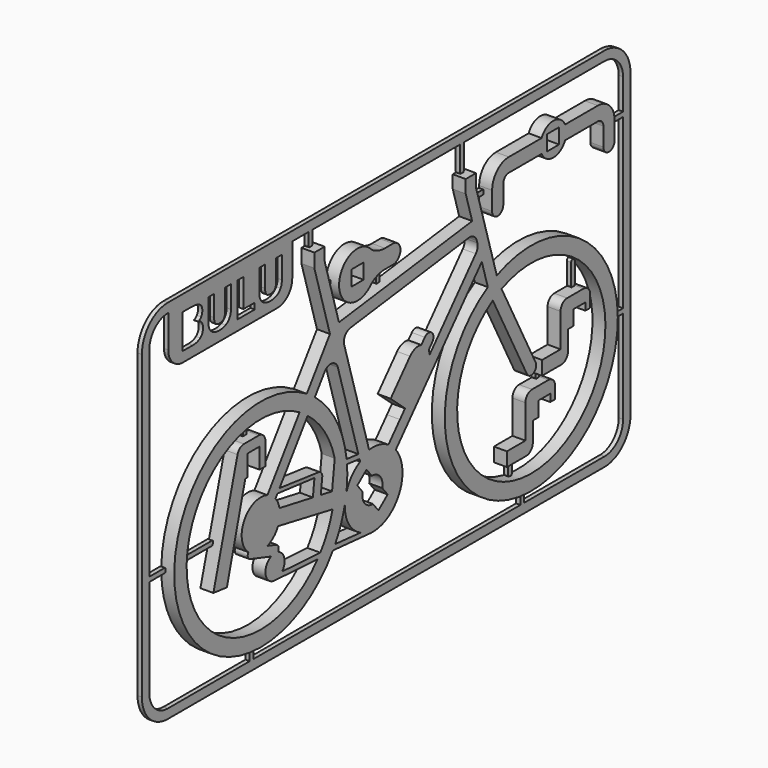
from build123d import *

# Parameters (mm, degrees)
F2_DEPTH = 2.8
F1_W     = 3.286
F1_H     = 3.286
F1_W_2   = 3.2
F1_H_2   = 3.2858568893
F3_DEPTH = 0.9333333333
F5_DEPTH = 0.9333333333
F7_DEPTH = 0.9333333333


# Not quite as in the source:
# - ends of sketch curves that miss each other by under 0.0002 mm in the source are joined
# - a feature names something its author has since deleted; it is built from what else it names


with BuildPart() as f2:
    # F1 (on Right) → F2 (new body)
    with BuildSketch(Plane.YZ):
        with BuildLine():
            Line((-32.7810810621, 40.0630099882), (-28.5785464468, 25.854345194))
            Line((-28.5785464468, 25.854345194), (-34.8295213879, 17.0517607704))
            ThreePointArc((-34.8295213879, 17.0517607704), (-70.0441528649, -7.6634310767), (-27.7561804721, -15.577871613))
            Line((-27.7561804721, -15.577871613), (-17.4309209468, -16.4342678025))
            ThreePointArc((-17.4309209468, -16.4342678025), (-17.421352009, -16.4349690955), (-17.4117713764, -16.4354866475))
            ThreePointArc((-17.4117713764, -16.4354866475), (-9.8783278177, -12.024945839), (-10.8100300989, -3.3452239002))
            Line((-10.8100300989, -3.3452239002), (12.3781786089, 22.9225390659))
            Line((12.3781786089, 22.9225390659), (13.9960358427, 17.4527707038))
            ThreePointArc((13.9960358427, 17.4527707038), (36.2440392418, -23.5369879191), (16.4146126558, 18.6758988393))
            Line((16.4146126558, 18.6758988393), (14.2536723845, 25.9817614853))
            ThreePointArc((14.2536723845, 25.9817614853), (14.2515405676, 25.989045047), (14.2493673209, 25.9963163545))
            Line((14.2493673209, 25.9963163545), (12.7777300944, 30.9717335764))
            Line((12.7777300944, 30.9717335764), (10.8173713638, 37.5995357396))
            Line((10.8173713638, 37.5995357396), (10.8173713638, 40.3995357399))
            Line((10.8173713638, 40.3995357399), (8.037018366, 40.3995357399))
            Line((8.037018366, 40.3995357399), (8.037018366, 37.5995357399))
            Line((8.037018366, 37.5995357399), (9.7773678827, 31.7155655707))
            Line((9.7773678827, 31.7155655707), (-26.1566620581, 27.0789083905))
            Line((-26.1566620581, 27.0789083905), (-30.0007321323, 40.2276701755))
            Line((-30.0007321323, 40.2276701755), (-30.0007321323, 43.0276701755))
            Line((-30.0007321323, 43.0276701755), (-32.7810810175, 43.0276701755))
            Line((-32.7810810175, 43.0276701755), (-32.7810810621, 40.0630099882))
        make_face()
        with BuildLine():
            ThreePointArc((-27.1589419206, -14.6239739066), (-25.6381564049, -11.5709515578), (-24.5785787783, -8.3288797973))
            ThreePointArc((-24.5785787783, -8.3288797973), (-23.4485868958, -12.4014570535), (-20.3032664054, -15.2245273988))
            Line((-20.3032664054, -15.2245273988), (-27.1589419206, -14.6239739066))
        make_face(mode=Mode.SUBTRACT)
        with BuildLine():
            Line((-36.7690909191, 14.3204708989), (-45.438959238, 2.1116157144))
            ThreePointArc((-45.438959238, 2.1116157144), (-51.679021575, -0.1114645339), (-50.5741858599, -6.6429116785))
            ThreePointArc((-50.5741858599, -6.6429116785), (-50.7001368643, -7.5358957288), (-50.0559554, -8.1670172786))
            Line((-50.0559554, -8.1670172786), (-44.4357401431, -9.9504751803))
            ThreePointArc((-44.4357401431, -9.9504751803), (-45.9475994843, -12.7053301629), (-43.682084094, -14.8830318549))
            Line((-43.682084094, -14.8830318549), (-43.4085644782, -14.8992046485))
            Line((-43.4085644782, -14.8992046485), (-31.9213599112, -15.5784253597))
            ThreePointArc((-31.9213599112, -15.5784253597), (-66.9726575865, -5.9191061127), (-36.7690909191, 14.3204708989))
        make_face(mode=Mode.SUBTRACT)
        with BuildLine():
            ThreePointArc((-45.417431414, -7.5410613439), (-43.7533998551, -6.5186996051), (-42.5893207169, -4.9505336974))
            Line((-42.5893207169, -4.9505336974), (-27.8742179451, -7.7233503042))
            ThreePointArc((-27.8742179451, -7.7233503042), (-29.1875288387, -11.3310895929), (-31.1661285889, -14.6213344633))
            Line((-31.1661285889, -14.6213344633), (-41.4453615912, -14.013539249))
            ThreePointArc((-41.4453615912, -14.013539249), (-40.8757428579, -11.7304415251), (-42.3931878811, -9.9320085072))
            Line((-42.3931878811, -9.9320085072), (-42.3931878811, -9.2324187691))
            ThreePointArc((-42.3931878811, -9.2324187691), (-42.5861622295, -8.6419628585), (-43.0905932927, -8.2794348124))
            Line((-43.0905932927, -8.2794348124), (-45.417431414, -7.5410613439))
        make_face(mode=Mode.SUBTRACT)
        with BuildLine():
            Line((-15.5088098858, -12.9576973057), (-16.9709924298, -11.149063212))
            ThreePointArc((-16.9709924298, -11.149063212), (-19.2224479888, -10.1072740955), (-19.7694541503, -7.6875301098))
            Line((-19.7694541503, -7.6875301098), (-21.2014292566, -5.9162608458))
            Line((-21.2014292566, -5.9162608458), (-18.7129342238, -3.9044476159))
            Line((-18.7129342238, -3.9044476159), (-17.2809591175, -5.67571688))
            ThreePointArc((-17.2809591175, -5.67571688), (-15.0295035586, -6.7175059964), (-14.4824973971, -9.1372499821))
            Line((-14.4824973971, -9.1372499821), (-13.0203148531, -10.9458840758))
            Line((-13.0203148531, -10.9458840758), (-15.5088098858, -12.9576973057))
        make_face(mode=Mode.SUBTRACT)
        with BuildLine():
            ThreePointArc((-20.4284332347, -1.7008787129), (-22.713034199, -3.5049348102), (-24.1327228009, -6.0462935497))
            ThreePointArc((-24.1327228009, -6.0462935497), (-23.9042746908, -3.4009611929), (-23.9777551737, -0.7467998497))
            Line((-23.9777551737, -0.7467998497), (-20.6010095051, -1.1174049345))
            Line((-20.6010095051, -1.1174049345), (-20.4284332347, -1.7008787129))
        make_face(mode=Mode.SUBTRACT)
        with BuildLine():
            ThreePointArc((-42.1876674295, -1.6755199445), (-42.5889328041, -0.4877747618), (-43.2651398515, 0.5679224243))
            Line((-43.2651398515, 0.5679224243), (-42.7367221094, 1.3120370351))
            Line((-42.7367221094, 1.3120370351), (-32.7536984043, 0.2163787562))
            Line((-32.7536984043, 0.2163787562), (-33.1812144267, -3.3188663768))
            Line((-33.1812144267, -3.3188663768), (-42.1876674295, -1.6755199445))
        make_face(mode=Mode.SUBTRACT)
        with BuildLine():
            Line((-31.6963693255, 0.8509632025), (-42.1651316758, 2.1169471643))
            Line((-42.1651316758, 2.1169471643), (-34.5952715328, 12.7767776084))
            ThreePointArc((-34.5952715328, 12.7767776084), (-29.9994401309, 7.8666759835), (-27.2914488726, 1.7105775773))
            Line((-27.2914488726, 1.7105775773), (-28.0136806178, -4.2617512446))
            Line((-28.0136806178, -4.2617512446), (-31.0443248868, -3.708770127))
            Line((-31.0443248868, -3.708770127), (-30.6536988323, -0.4785780739))
            ThreePointArc((-30.6536988323, -0.4785780739), (-30.8996770647, 0.402136694), (-31.6963693255, 0.8509632025))
        make_face(mode=Mode.SUBTRACT)
        with BuildLine():
            ThreePointArc((24.5326127574, -3.3329199604), (26.3299626073, -3.9019308276), (26.8989734744, -2.1045809777))
            Line((26.8989734744, -2.1045809777), (17.7069262182, 15.603641135))
            ThreePointArc((17.7069262182, 15.603641135), (34.9283354862, -20.4664558462), (15.3405655012, 14.3753021523))
            Line((15.3405655012, 14.3753021523), (24.5326127574, -3.3329199604))
        make_face(mode=Mode.SUBTRACT)
        with BuildLine():
            ThreePointArc((-29.9983734724, 19.2501011531), (-28.0396469956, 20.0648164886), (-26.4504948685, 18.6594816511))
            Line((-26.4504948685, 18.6594816511), (-20.9085424497, -0.0776477954))
            Line((-20.9085424497, -0.0776477954), (-24.0866021245, 0.2711510752))
            ThreePointArc((-24.0866021245, 0.2711510752), (-26.8907561473, 8.722170153), (-32.6557020014, 15.5080674802))
            Line((-32.6557020014, 15.5080674802), (-29.9983734724, 19.2501011531))
        make_face(mode=Mode.SUBTRACT)
        with BuildLine():
            Line((-18.0250834345, -0.4262562289), (-24.7288519992, 22.2389292241))
            ThreePointArc((-24.7288519992, 22.2389292241), (-24.4867438443, 23.8976541842), (-23.0672336955, 24.7892683327))
            Line((-23.0672336955, 24.7892683327), (8.8532049047, 28.9080418475))
            ThreePointArc((8.8532049047, 28.9080418475), (10.2006691115, 28.6002630517), (11.0266106326, 27.4920175106))
            Line((11.0266106326, 27.4920175106), (11.1717955661, 27.0011658215))
            ThreePointArc((11.1717955661, 27.0011658215), (11.2066686934, 26.0018903312), (10.7533788193, 25.1106575162))
            Line((10.7533788193, 25.1106575162), (-1.7245508843, 10.9755725718))
            ThreePointArc((-1.7245508843, 10.9755725718), (-1.7897327542, 11.4952481661), (-1.9443174541, 11.9956629641))
            Line((-1.9443174541, 11.9956629641), (-0.9945827645, 13.0715289795))
            ThreePointArc((-0.9945827646, 13.0715289795), (-1.1117489129, 14.9531537943), (-2.9933737277, 14.8359876459))
            Line((-2.9933737277, 14.8359876459), (-3.9431084172, 13.7601216304))
            ThreePointArc((-3.9431084172, 13.7601216304), (-5.5866841115, 13.7356227774), (-6.9705428385, 12.8485623057))
            Line((-6.9705428385, 12.8485623057), (-12.2077076552, 6.9158658319))
            Line((-12.2077076552, 6.9158658319), (-8.3300521573, 3.4928151103))
            Line((-8.3300521573, 3.4928151103), (-9.6983886135, 1.9427541226))
            Line((-9.6983886135, 1.9427541226), (-12.8088210603, -1.5807652347))
            ThreePointArc((-12.8088210603, -1.5807652347), (-15.3182270596, -0.5574540272), (-18.0250834345, -0.4262562289))
        make_face(mode=Mode.SUBTRACT)
    extrude(amount=F2_DEPTH)



with BuildPart() as f2b:
    # F1 (on Right) → F2, piece 2 (new body)
    with BuildSketch(Plane.YZ):
        with BuildLine():
            Line((26.1350085661, -17.0272199881), (26.1350085661, -12.8250569627))
            Line((26.1350085661, -12.8250569627), (27.6350085661, -12.8250569627))
            Line((27.6350085661, -12.8250569627), (27.6350085661, -9.6250569627))
            Line((27.6350085661, -9.6250569627), (30.8350085661, -9.6250569627))
            Line((30.8350085661, -9.6250569627), (30.8350085661, -11.2250569627))
            Line((30.8350085661, -11.2250569627), (32.1350085661, -11.2250569627))
            Line((32.1350085661, -11.2250569627), (32.1350085661, -8.6228939372))
            ThreePointArc((32.1350085661, -8.6228939372), (31.6084343077, -7.351631221), (30.3371715916, -6.8250569627))
            Line((30.3371715916, -6.8250569627), (26.1350085661, -6.8250569627))
            Line((26.1350085661, -6.8250569627), (25.9328455406, -6.8250569627))
            ThreePointArc((25.9328455406, -6.8250569627), (24.6615828245, -7.351631221), (24.1350085661, -8.6228939372))
            Line((24.1350085661, -8.6228939372), (24.1350085661, -15.8250569627))
            Line((24.1350085661, -15.8250569627), (19.1350085661, -15.8250569627))
            Line((19.1350085661, -15.8250569627), (19.1350085661, -18.8250569627))
            Line((19.1350085661, -18.8250569627), (24.3371715916, -18.8250569627))
            ThreePointArc((24.3371715916, -18.8250569627), (25.6084343077, -18.2984827043), (26.1350085661, -17.0272199881))
        make_face()
    extrude(amount=F2_DEPTH)


with BuildPart() as f2c:
    # F1 (on Right) → F2, piece 3 (new body)
    with BuildSketch(Plane.YZ):
        with BuildLine():
            Line((-47.7713023129, 14.3973374015), (-51.7613397022, 14.3973374015))
            ThreePointArc((-51.7613397022, 14.3973374015), (-52.8518038089, 14.0305013357), (-53.496568146, 13.077632186))
            Line((-53.496568146, 13.077632186), (-60.0158057756, -10.5528221893))
            Line((-60.0158057756, -10.5528221893), (-56.367214369, -10.9714387513))
            Line((-56.367214369, -10.9714387513), (-51.4058386912, 7.6636058447))
            Line((-51.4058386912, 7.6636058447), (-50.7571436434, 7.6636058447))
            Line((-50.7571436434, 7.6636058447), (-50.7571436434, 12.2000958209))
            Line((-50.7571436434, 12.2000958209), (-47.5571436434, 12.2000958209))
            Line((-47.5571436434, 12.2000958209), (-47.5571436434, 7.799523944))
            Line((-47.5571436434, 7.799523944), (-45.9734653383, 7.799523944))
            Line((-45.9734653383, 7.799523944), (-45.9734653383, 12.599500427))
            ThreePointArc((-45.9734653383, 12.599500427), (-46.5000395967, 13.8707631432), (-47.7713023129, 14.3973374015))
        make_face()
    extrude(amount=F2_DEPTH)


with BuildPart() as f2d:
    # F1 (on Right) → F2, piece 4 (new body)
    with BuildSketch(Plane.YZ):
        with BuildLine():
            ThreePointArc((-11.5660707645, 32.1164598398), (-9.5660707645, 34.1164598398), (-11.5660707645, 36.1164598398))
            Line((-11.5660707645, 36.1164598398), (-13.7510611544, 36.1164598398))
            ThreePointArc((-13.7510611544, 36.1164598398), (-15.6803701734, 36.4351072976), (-17.4047560543, 37.35720427))
            ThreePointArc((-17.4047560543, 37.35720427), (-26.1140103212, 34.1164598398), (-17.4047560543, 30.8757154096))
            ThreePointArc((-17.4047560543, 30.8757154096), (-15.6803701734, 31.7978123821), (-13.7510611544, 32.1164598398))
            Line((-13.7510611544, 32.1164598398), (-11.5660707645, 32.1164598398))
        make_face()
        with Locations((-21.1564369343, 34.1164598398)):
            Rectangle(F1_W, F1_H, mode=Mode.SUBTRACT)
    extrude(amount=F2_DEPTH)


with BuildPart() as f2e:
    # F1 (on Right) → F2, piece 5 (new body)
    with BuildSketch(Plane.YZ):
        with BuildLine():
            ThreePointArc((15.1628487238, 31.3657282359), (16.6628487238, 29.8657282359), (18.1628487238, 31.3657282359))
            Line((18.1628487238, 31.3657282359), (18.1628487238, 35.3657282359))
            ThreePointArc((18.1628487238, 35.3657282359), (18.602188552, 36.4263884077), (19.6628487238, 36.8657282359))
            Line((19.6628487238, 36.8657282359), (28.5005710636, 36.8657282359))
            ThreePointArc((28.5005710636, 36.8657282359), (31.6628487238, 34.8657282359), (34.825126384, 36.8657282359))
            Line((34.825126384, 36.8657282359), (43.6628487238, 36.8657282359))
            ThreePointArc((43.6628487238, 36.8657282359), (44.7235088956, 36.4263884077), (45.1628487238, 35.3657282359))
            Line((45.1628487238, 35.3657282359), (45.1628487238, 31.3657282359))
            ThreePointArc((45.1628487238, 31.3657282359), (46.6628487238, 29.8657282359), (48.1628487238, 31.3657282359))
            Line((48.1628487238, 31.3657282359), (48.1628487238, 35.3657282359))
            ThreePointArc((48.1628487238, 35.3657282359), (46.8448292391, 38.5477087513), (43.6628487238, 39.8657282359))
            Line((43.6628487238, 39.8657282359), (34.825126384, 39.8657282359))
            ThreePointArc((34.825126384, 39.8657282359), (31.6628487238, 41.8657282359), (28.5005710636, 39.8657282359))
            Line((28.5005710636, 39.8657282359), (19.6628487238, 39.8657282359))
            ThreePointArc((19.6628487238, 39.8657282359), (16.4808682084, 38.5477087513), (15.1628487238, 35.3657282359))
            Line((15.1628487238, 35.3657282359), (15.1628487238, 31.3657282359))
        make_face()
        with Locations((31.6199202791, 38.3657282359)):
            Rectangle(F1_W_2, F1_H_2, mode=Mode.SUBTRACT)
    extrude(amount=F2_DEPTH)


with BuildPart() as f2f:
    # F1 (on Right) → F2, piece 6 (new body)
    with BuildSketch(Plane.YZ):
        with BuildLine():
            Line((39.8146519543, 6.6714825634), (35.6124889288, 6.6714825634))
            Line((35.6124889288, 6.6714825634), (35.4103259033, 6.6714825634))
            ThreePointArc((35.4103259033, 6.6714825634), (34.1390631872, 6.144908305), (33.6124889288, 4.8736455889))
            Line((33.6124889288, 4.8736455889), (33.6124889288, -2.3285174366))
            Line((33.6124889288, -2.3285174366), (28.6124889288, -2.3285174366))
            Line((28.6124889288, -2.3285174366), (28.6124889288, -5.3285174366))
            Line((28.6124889288, -5.3285174366), (33.8146519543, -5.3285174366))
            ThreePointArc((33.8146519543, -5.3285174366), (35.0859146704, -4.8019431782), (35.6124889288, -3.5306804621))
            Line((35.6124889288, -3.5306804621), (35.6124889288, 0.6714825634))
            Line((35.6124889288, 0.6714825634), (37.1124889288, 0.6714825634))
            Line((37.1124889288, 0.6714825634), (37.1124889288, 3.8714825634))
            Line((37.1124889288, 3.8714825634), (40.3124889288, 3.8714825634))
            Line((40.3124889288, 3.8714825634), (40.3124889288, 2.2714825634))
            Line((40.3124889288, 2.2714825634), (41.6124889288, 2.2714825634))
            Line((41.6124889288, 2.2714825634), (41.6124889288, 4.8736455889))
            ThreePointArc((41.6124889288, 4.8736455889), (41.0859146704, 6.144908305), (39.8146519543, 6.6714825634))
        make_face()
    extrude(amount=F2_DEPTH)


with BuildPart() as f3:
    # F1 (on Right) → F3 (new body)
    with BuildSketch(Plane.YZ):
        with BuildLine():
            ThreePointArc((-76.9647278786, -24.0477662427), (-74.9144753469, -28.9975137111), (-69.9647278786, -31.0477662427))
            Line((-69.9647278786, -31.0477662427), (47.795983851, -31.0477662427))
            ThreePointArc((47.795983851, -31.0477662427), (52.7457313193, -28.9975137111), (54.795983851, -24.0477662427))
            Line((54.795983851, -24.0477662427), (54.795983851, 41.0276701755))
            ThreePointArc((54.795983851, 41.0276701755), (52.7457313193, 45.9774176438), (47.795983851, 48.0276701755))
            Line((47.795983851, 48.0276701755), (-69.9647278786, 48.0276701755))
            ThreePointArc((-69.9647278786, 48.0276701755), (-74.9144753469, 45.9774176438), (-76.9647278786, 41.0276701755))
            Line((-76.9647278786, 41.0276701755), (-76.9647278786, -24.0477662427))
        make_face()
        with BuildLine():
            Line((47.795983851, -29.0477662427), (-69.9647278786, -29.0477662427))
            ThreePointArc((-69.9647278786, -29.0477662427), (-73.5002617845, -27.5833001487), (-74.9647278786, -24.0477662427))
            Line((-74.9647278786, -24.0477662427), (-74.9647278786, 41.0276701755))
            ThreePointArc((-74.9647278786, 41.0276701755), (-73.5002617845, 44.5632040814), (-69.9647278786, 46.0276701755))
            Line((-69.9647278786, 46.0276701755), (-64.4556283951, 46.0276701755))
            Line((-64.4556283951, 46.0276701755), (-38.3469462395, 46.0276701755))
            Line((-38.3469462395, 46.0276701755), (47.795983851, 46.0276701755))
            ThreePointArc((47.795983851, 46.0276701755), (51.3315177569, 44.5632040814), (52.795983851, 41.0276701755))
            Line((52.795983851, 41.0276701755), (52.795983851, -24.0477662427))
            ThreePointArc((52.795983851, -24.0477662427), (51.3315177569, -27.5833001487), (47.795983851, -29.0477662427))
        make_face(mode=Mode.SUBTRACT)
    extrude(amount=F3_DEPTH)


with BuildPart() as f2_1:
    add(f2.part)

    add(f2b.part)  # F5 merges F2b

    add(f2c.part)  # F5 merges F2c

    add(f2d.part)  # F5 merges F2d

    add(f2e.part)  # F5 merges F2e

    add(f2f.part)  # F5 merges F2f

    add(f3.part)  # F5 merges F3
    # F4 (on Right) → F5 (join)
    with BuildSketch(Plane.YZ):
        with BuildLine():
            ThreePointArc((-49.7433960476, 14.0407793284), (-49.2433960476, 13.5407793284), (-48.7433960476, 14.0407793284))
            Line((-48.7433960476, 14.0407793284), (-48.7433960476, 16.7634686467))
            ThreePointArc((-48.7433960476, 16.7634686467), (-49.2433960476, 17.2634686467), (-49.7433960476, 16.7634686467))
            Line((-49.7433960476, 16.7634686467), (-49.7433960476, 14.0407793284))
        make_face()
        with BuildLine():
            ThreePointArc((-66.8206203722, -2.0058723694), (-67.3206203722, -2.5058723694), (-66.8206203722, -3.0058723694))
            Line((-66.8206203722, -3.0058723694), (-58.1512004137, -3.0058723694))
            ThreePointArc((-58.1512004137, -3.0058723694), (-57.6512004137, -2.5058723694), (-58.1512004137, -2.0058723694))
            Line((-58.1512004137, -2.0058723694), (-66.8206203722, -2.0058723694))
        make_face()
        with BuildLine():
            ThreePointArc((-70.9232541835, -3.0058723694), (-70.4232541835, -2.5058723694), (-70.9232541835, -2.0058723694))
            Line((-70.9232541835, -2.0058723694), (-74.9647278786, -2.0058723694))
            ThreePointArc((-74.9647278786, -2.0058723694), (-75.4647278786, -2.5058723694), (-74.9647278786, -3.0058723694))
            Line((-74.9647278786, -3.0058723694), (-70.9232541835, -3.0058723694))
        make_face()
        with BuildLine():
            ThreePointArc((-31.9633883536, 43.3622263372), (-31.4633883536, 42.8622263372), (-30.9633883536, 43.3622263372))
            Line((-30.9633883536, 43.3622263372), (-30.9633883536, 46.4626848698))
            ThreePointArc((-30.9633883536, 46.4626848698), (-31.4633883536, 46.9626848698), (-31.9633883536, 46.4626848698))
            Line((-31.9633883536, 46.4626848698), (-31.9633883536, 43.3622263372))
        make_face()
        with BuildLine():
            ThreePointArc((-27.9091558336, 34.6210477054), (-28.4091558336, 34.1210477054), (-27.9091558336, 33.6210477054))
            Line((-27.9091558336, 33.6210477054), (-26.4964278766, 33.6210477054))
            ThreePointArc((-26.4964278766, 33.6210477054), (-25.9964278766, 34.1210477054), (-26.4964278766, 34.6210477054))
            Line((-26.4964278766, 34.6210477054), (-27.9091558336, 34.6210477054))
        make_face()
        with BuildLine():
            Line((-13.8486790583, 31.6781923175), (-13.8486790583, 29.1007384658))
            ThreePointArc((-13.8486790583, 29.1007384658), (-13.3486790583, 28.6007384658), (-12.8486790583, 29.1007384658))
            Line((-12.8486790583, 29.1007384658), (-12.8486790583, 31.6781923175))
            ThreePointArc((-12.8486790583, 31.6781923175), (-13.3486790583, 32.1781923175), (-13.8486790583, 31.6781923175))
        make_face()
        with BuildLine():
            Line((8.8458192423, 46.0585150868), (8.8458192423, 40.6653936952))
            ThreePointArc((8.8458192423, 40.6653936952), (9.3458192423, 40.1653936952), (9.8458192423, 40.6653936952))
            Line((9.8458192423, 40.6653936952), (9.8458192423, 46.0585150868))
            ThreePointArc((9.8458192423, 46.0585150868), (9.3458192423, 46.5585150868), (8.8458192423, 46.0585150868))
        make_face()
        with BuildLine():
            ThreePointArc((11.9448483718, 34.9700198621), (11.4448483718, 34.4700198621), (11.9448483718, 33.9700198621))
            Line((11.9448483718, 33.9700198621), (14.8754121757, 33.9700198621))
            ThreePointArc((14.8754121757, 33.9700198621), (15.3754121757, 34.4700198621), (14.8754121757, 34.9700198621))
            Line((14.8754121757, 34.9700198621), (11.9448483718, 34.9700198621))
        make_face()
        with BuildLine():
            ThreePointArc((48.4550757053, 34.3975656778), (47.9550757053, 33.8975656778), (48.4550757053, 33.3975656778))
            Line((48.4550757053, 33.3975656778), (52.9664561174, 33.3975656778))
            ThreePointArc((52.9664561174, 33.3975656778), (53.4664561174, 33.8975656778), (52.9664561174, 34.3975656778))
            Line((52.9664561174, 34.3975656778), (48.4550757053, 34.3975656778))
        make_face()
        with BuildLine():
            Line((38.7966382205, 11.4560816437), (38.7966382205, 6.9804331288))
            ThreePointArc((38.7966382205, 6.9804331288), (39.2966382205, 6.4804331288), (39.7966382205, 6.9804331288))
            Line((39.7966382205, 6.9804331288), (39.7966382205, 11.4560816437))
            ThreePointArc((39.7966382205, 11.4560816437), (39.2966382205, 11.9560816437), (38.7966382205, 11.4560816437))
        make_face()
        with BuildLine():
            Line((49.2580496178, -3.9376585865), (53.1618170887, -3.9376585865))
            ThreePointArc((53.1618170887, -3.9376585865), (53.6618170887, -3.4376585865), (53.1618170887, -2.9376585865))
            Line((53.1618170887, -2.9376585865), (49.2580496178, -2.9376585865))
            ThreePointArc((49.2580496178, -2.9376585865), (48.7580496178, -3.4376585865), (49.2580496178, -3.9376585865))
        make_face()
        with BuildLine():
            Line((29.1594016254, -5.6311495136), (29.1594016254, -6.4238952473))
            ThreePointArc((29.1594016254, -6.4238952473), (29.6594016254, -6.9238952473), (30.1594016254, -6.4238952473))
            Line((30.1594016254, -6.4238952473), (30.1594016254, -5.6311495136))
            ThreePointArc((30.1594016254, -5.6311495136), (29.6594016254, -5.1311495136), (29.1594016254, -5.6311495136))
        make_face()
        with BuildLine():
            Line((21.8041344434, -19.2048698664), (21.8041344434, -22.0675207675))
            ThreePointArc((21.8041344434, -22.0675207675), (22.3041344434, -22.5675207675), (22.8041344434, -22.0675207675))
            Line((22.8041344434, -22.0675207675), (22.8041344434, -19.2048698664))
            ThreePointArc((22.8041344434, -19.2048698664), (22.3041344434, -18.7048698664), (21.8041344434, -19.2048698664))
        make_face()
        with BuildLine():
            Line((25.1091188639, -26.3297744095), (25.1091188639, -29.1924253106))
            ThreePointArc((25.1091188639, -29.1924253106), (25.6091188639, -29.6924253106), (26.1091188639, -29.1924253106))
            Line((26.1091188639, -29.1924253106), (26.1091188639, -26.3297744095))
            ThreePointArc((26.1091188639, -26.3297744095), (25.6091188639, -25.8297744095), (25.1091188639, -26.3297744095))
        make_face()
        with BuildLine():
            Line((-47.8730191588, -26.3541825116), (-47.8730191588, -29.2168334126))
            ThreePointArc((-47.8730191588, -29.2168334126), (-47.3730191588, -29.7168334126), (-46.8730191588, -29.2168334126))
            Line((-46.8730191588, -29.2168334126), (-46.8730191588, -26.3541825116))
            ThreePointArc((-46.8730191588, -26.3541825116), (-47.3730191588, -25.8541825116), (-47.8730191588, -26.3541825116))
        make_face()
    extrude(amount=F5_DEPTH)

    # F6 (on Right) → F7 (join, through all)
    with BuildSketch(Plane.YZ):
        with BuildLine():
            Line((-36.4059554021, 46.0276701755), (-69.8416978121, 46.0276701755))
            Line((-69.8416978121, 46.0276701755), (-69.8416978121, 39.0079783506))
            ThreePointArc((-69.8416978121, 39.0079783506), (-68.6701249368, 36.1795512258), (-65.8416978121, 35.0079783506))
            Line((-65.8416978121, 35.0079783506), (-40.4059554021, 35.0079783506))
            ThreePointArc((-40.4059554021, 35.0079783506), (-37.5775282774, 36.1795512258), (-36.4059554021, 39.0079783506))
            Line((-36.4059554021, 39.0079783506), (-36.4059554021, 46.0276701755))
        make_face()
        with BuildLine():
            Line((-65.9799783332, 37.2014082968), (-65.9799783332, 44.6279588747))
            Line((-65.9799783332, 44.6279588747), (-63.6686290398, 44.6279588747))
            add(Edge.make_bspline(
                [(-63.6686290398, 44.6279588747), (-62.0887193961, 44.6279588747), (-61.3751593822, 44.1785298454)],
                knots=[0, 0, 0, 1, 1, 1], degree=2))
            add(Edge.make_bspline(
                [(-61.3751593822, 44.1785298454), (-60.6615993683, 43.7291008162), (-60.6615993683, 42.7489716854)],
                knots=[0, 0, 0, 1, 1, 1], degree=2))
            add(Edge.make_bspline(
                [(-60.6615993683, 42.7489716854), (-60.6615993683, 42.0825488933), (-60.9736802855, 41.6558757643)],
                knots=[0, 0, 0, 1, 1, 1], degree=2))
            add(Edge.make_bspline(
                [(-60.9736802855, 41.6558757643), (-61.2857612028, 41.2292026352), (-61.8042706434, 41.1430552987)],
                knots=[0, 0, 0, 1, 1, 1], degree=2))
            Line((-61.8042706434, 41.1430552987), (-61.8042706434, 41.0926672339))
            add(Edge.make_bspline(
                [(-61.8042706434, 41.0926672339), (-61.0988377367, 40.9350013538), (-60.7859441087, 40.5034519604)],
                knots=[0, 0, 0, 1, 1, 1], degree=2))
            add(Edge.make_bspline(
                [(-60.7859441087, 40.5034519604), (-60.4730504807, 40.071902567), (-60.4730504807, 39.3550917102)],
                knots=[0, 0, 0, 1, 1, 1], degree=2))
            add(Edge.make_bspline(
                [(-60.4730504807, 39.3550917102), (-60.4730504807, 38.3392033077), (-61.2077409735, 37.7703058022)],
                knots=[0, 0, 0, 1, 1, 1], degree=2))
            add(Edge.make_bspline(
                [(-61.2077409735, 37.7703058022), (-61.9424314662, 37.2014082968), (-63.2021330853, 37.2014082968)],
                knots=[0, 0, 0, 1, 1, 1], degree=2))
            Line((-63.2021330853, 37.2014082968), (-65.9799783332, 37.2014082968))
        make_face(mode=Mode.SUBTRACT)
        with BuildLine():
            Line((-54.5158808883, 44.6279588747), (-52.9457237733, 44.6279588747))
            Line((-52.9457237733, 44.6279588747), (-52.9457237733, 39.8232130861))
            add(Edge.make_bspline(
                [(-52.9457237733, 39.8232130861), (-52.9457237733, 38.999124414), (-53.3138817304, 38.3798388438)],
                knots=[0, 0, 0, 1, 1, 1], degree=2))
            add(Edge.make_bspline(
                [(-53.3138817304, 38.3798388438), (-53.6820396875, 37.7605532736), (-54.3785327763, 37.4297800097)],
                knots=[0, 0, 0, 1, 1, 1], degree=2))
            add(Edge.make_bspline(
                [(-54.3785327763, 37.4297800097), (-55.075025865, 37.0990067458), (-56.0242719884, 37.0990067458)],
                knots=[0, 0, 0, 1, 1, 1], degree=2))
            add(Edge.make_bspline(
                [(-56.0242719884, 37.0990067458), (-57.4562682806, 37.0990067458), (-58.2486612346, 37.8336972386)],
                knots=[0, 0, 0, 1, 1, 1], degree=2))
            add(Edge.make_bspline(
                [(-58.2486612346, 37.8336972386), (-59.0410541885, 38.5683877313), (-59.0410541885, 39.8427181434)],
                knots=[0, 0, 0, 1, 1, 1], degree=2))
            Line((-59.0410541885, 39.8427181434), (-59.0410541885, 44.6279588747))
            Line((-59.0410541885, 44.6279588747), (-57.472522495, 44.6279588747))
            Line((-57.472522495, 44.6279588747), (-57.472522495, 40.0816550957))
            add(Edge.make_bspline(
                [(-57.472522495, 40.0816550957), (-57.472522495, 39.2234325732), (-57.1271204382, 38.8219534765)],
                knots=[0, 0, 0, 1, 1, 1], degree=2))
            add(Edge.make_bspline(
                [(-57.1271204382, 38.8219534765), (-56.7817183813, 38.4204743799), (-55.9836364523, 38.4204743799)],
                knots=[0, 0, 0, 1, 1, 1], degree=2))
            add(Edge.make_bspline(
                [(-55.9836364523, 38.4204743799), (-55.2115612663, 38.4204743799), (-54.8637210773, 38.8243916087)],
                knots=[0, 0, 0, 1, 1, 1], degree=2))
            add(Edge.make_bspline(
                [(-54.8637210773, 38.8243916087), (-54.5158808883, 39.2283088376), (-54.5158808883, 40.0914076244)],
                knots=[0, 0, 0, 1, 1, 1], degree=2))
            Line((-54.5158808883, 40.0914076244), (-54.5158808883, 44.6279588747))
        make_face(mode=Mode.SUBTRACT)
        Polygon((-46.5399378623, 37.2014082968), (-51.1268771774, 37.2014082968), (-51.1268771774, 44.6279588747), (-49.5518437981, 44.6279588747), (-49.5518437981, 38.5017454521), (-46.5399378623, 38.5017454521), align=None, mode=Mode.SUBTRACT)
        with BuildLine():
            Line((-40.7745680002, 44.6279588747), (-39.2044108853, 44.6279588747))
            Line((-39.2044108853, 44.6279588747), (-39.2044108853, 39.8232130861))
            add(Edge.make_bspline(
                [(-39.2044108853, 39.8232130861), (-39.2044108853, 38.999124414), (-39.5725688423, 38.3798388438)],
                knots=[0, 0, 0, 1, 1, 1], degree=2))
            add(Edge.make_bspline(
                [(-39.5725688423, 38.3798388438), (-39.9407267994, 37.7605532736), (-40.6372198882, 37.4297800097)],
                knots=[0, 0, 0, 1, 1, 1], degree=2))
            add(Edge.make_bspline(
                [(-40.6372198882, 37.4297800097), (-41.333712977, 37.0990067458), (-42.2829591003, 37.0990067458)],
                knots=[0, 0, 0, 1, 1, 1], degree=2))
            add(Edge.make_bspline(
                [(-42.2829591003, 37.0990067458), (-43.7149553925, 37.0990067458), (-44.5073483465, 37.8336972386)],
                knots=[0, 0, 0, 1, 1, 1], degree=2))
            add(Edge.make_bspline(
                [(-44.5073483465, 37.8336972386), (-45.2997413005, 38.5683877313), (-45.2997413005, 39.8427181434)],
                knots=[0, 0, 0, 1, 1, 1], degree=2))
            Line((-45.2997413005, 39.8427181434), (-45.2997413005, 44.6279588747))
            Line((-45.2997413005, 44.6279588747), (-43.731209607, 44.6279588747))
            Line((-43.731209607, 44.6279588747), (-43.731209607, 40.0816550957))
            add(Edge.make_bspline(
                [(-43.731209607, 40.0816550957), (-43.731209607, 39.2234325732), (-43.3858075501, 38.8219534765)],
                knots=[0, 0, 0, 1, 1, 1], degree=2))
            add(Edge.make_bspline(
                [(-43.3858075501, 38.8219534765), (-43.0404054932, 38.4204743799), (-42.2423235642, 38.4204743799)],
                knots=[0, 0, 0, 1, 1, 1], degree=2))
            add(Edge.make_bspline(
                [(-42.2423235642, 38.4204743799), (-41.4702483783, 38.4204743799), (-41.1224081892, 38.8243916087)],
                knots=[0, 0, 0, 1, 1, 1], degree=2))
            add(Edge.make_bspline(
                [(-41.1224081892, 38.8243916087), (-40.7745680002, 39.2283088376), (-40.7745680002, 40.0914076244)],
                knots=[0, 0, 0, 1, 1, 1], degree=2))
            Line((-40.7745680002, 40.0914076244), (-40.7745680002, 44.6279588747))
        make_face(mode=Mode.SUBTRACT)
    extrude(amount=F7_DEPTH)


solid = f2_1.part
